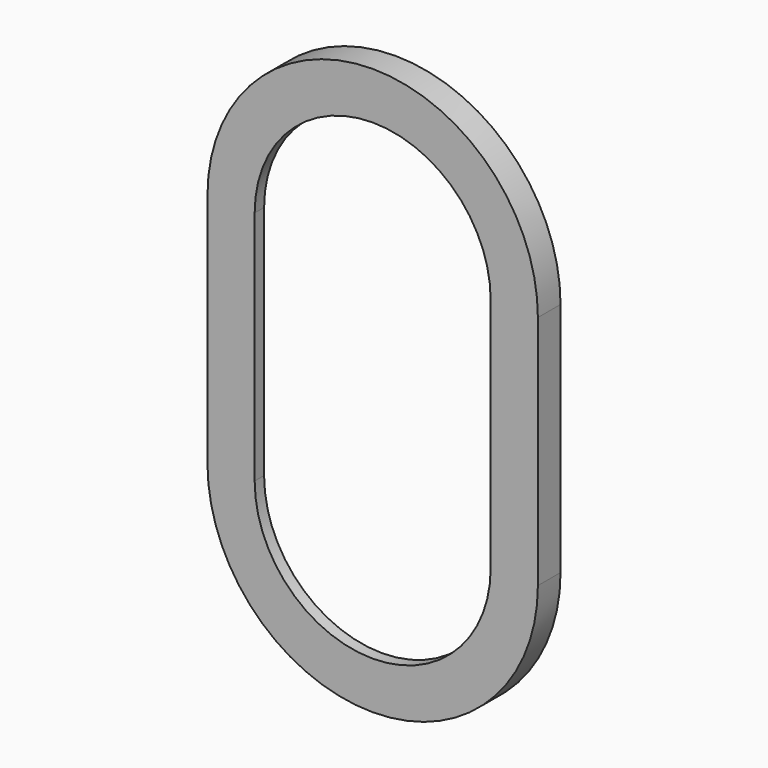
from build123d import *

# Parameters (mm, degrees)
F1_DEPTH = 12
F2_DEPTH = 7


# Not quite as in the source:
# - a feature of the source that left no trace in its solid (it failed there, or was rolled back) is left out


with BuildPart() as f1:
    # F0 (on Front) → F1 (new body)
    with BuildSketch(Plane.XZ):
        with BuildLine():
            Line((70, 130), (70, 230))
            ThreePointArc((70, 230), (0, 300), (-70, 230))
            Line((-70, 230), (-70, 130))
            ThreePointArc((-70, 130), (0, 60), (70, 130))
        make_face()
        with BuildLine():
            Line((-65, 130), (-65, 230))
            ThreePointArc((-65, 230), (0, 295), (65, 230))
            Line((65, 230), (65, 130))
            ThreePointArc((65, 130), (0, 65), (-65, 130))
        make_face(mode=Mode.SUBTRACT)
        with BuildLine():
            ThreePointArc((65, 230), (0, 295), (-65, 230))
            Line((-65, 230), (-65, 130))
            ThreePointArc((-65, 130), (0, 65), (65, 130))
            Line((65, 130), (65, 230))
        make_face()
        with BuildLine():
            Line((-50, 130), (-50, 230))
            ThreePointArc((-50, 230), (0, 280), (50, 230))
            Line((50, 230), (50, 130))
            ThreePointArc((50, 130), (0, 80), (-50, 130))
        make_face(mode=Mode.SUBTRACT)
    extrude(amount=F1_DEPTH)

    # F0 (on Front) → F2 (cut)
    with BuildSketch(Plane.XZ):
        with BuildLine():
            ThreePointArc((65, 230), (0, 295), (-65, 230))
            Line((-65, 230), (-65, 130))
            ThreePointArc((-65, 130), (0, 65), (65, 130))
            Line((65, 130), (65, 230))
        make_face()
        with BuildLine():
            Line((-50, 130), (-50, 230))
            ThreePointArc((-50, 230), (0, 280), (50, 230))
            Line((50, 230), (50, 130))
            ThreePointArc((50, 130), (0, 80), (-50, 130))
        make_face(mode=Mode.SUBTRACT)
    extrude(amount=F2_DEPTH, mode=Mode.SUBTRACT)


solid = f1.part
